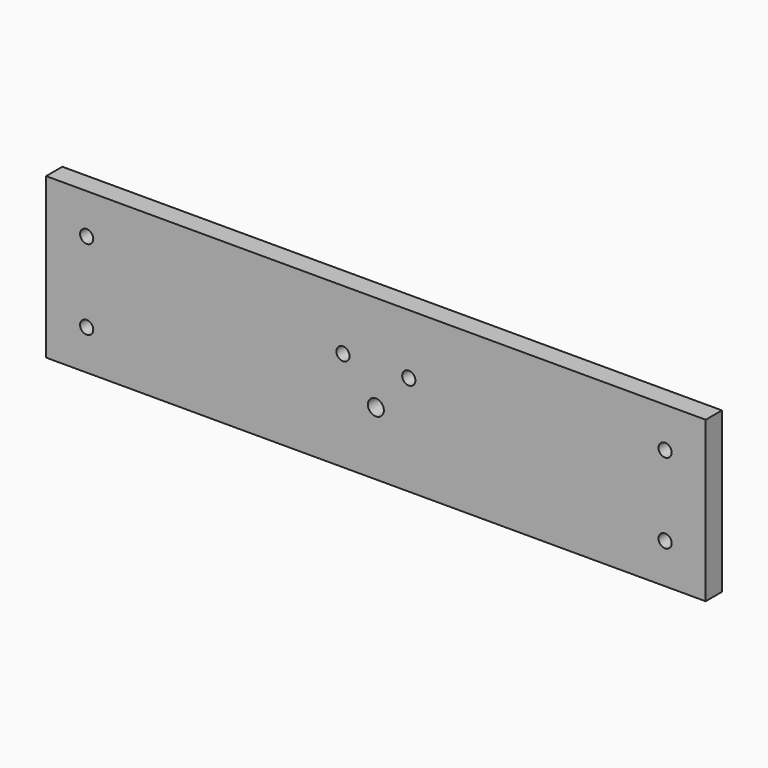
from build123d import *

# Parameters (mm, degrees)
F0_W     = 412.7
F0_H     = 100
F0_R     = 4.125
F0_R_2   = 5
F1_DEPTH = 12.7


# Not quite as in the source:
# - a length typed as a fraction of an inch, garbled in the dataset ("3 / 203.2 mm" for 3/8 in), is restored


with BuildPart() as f1:
    # F0 (on Front) → F1 (new body)
    with BuildSketch(Plane.XZ):
        with Locations((0, 7.472498)):
            Rectangle(F0_W, F0_H)
        with Locations((-180.95, -17.527502)):
            Circle(F0_R, mode=Mode.SUBTRACT)
        with Locations((0, -2.829017)):
            Circle(F0_R_2, mode=Mode.SUBTRACT)
        with Locations((180.95, -17.527502)):
            Circle(F0_R, mode=Mode.SUBTRACT)
        with Locations((-20.590066, 20.006112)):
            Circle(F0_R, mode=Mode.SUBTRACT)
        with Locations((-180.95, 32.472498)):
            Circle(F0_R, mode=Mode.SUBTRACT)
        with Locations((20.590066, 20.006112)):
            Circle(F0_R, mode=Mode.SUBTRACT)
        with Locations((180.95, 32.472498)):
            Circle(F0_R, mode=Mode.SUBTRACT)
    extrude(amount=F1_DEPTH)


solid = f1.part
